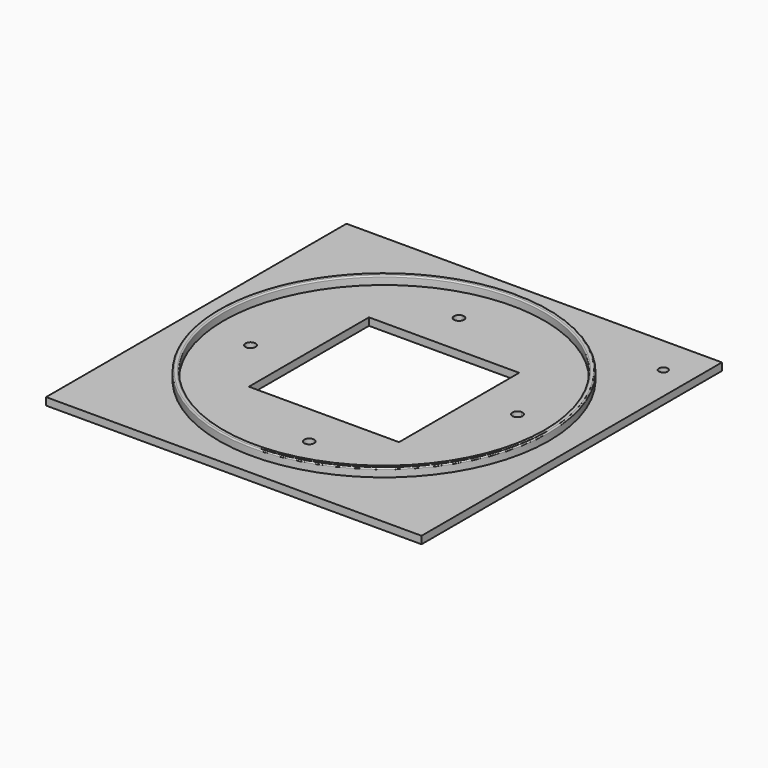
from build123d import *

# Parameters (mm, degrees)
F0_W     = 150
F0_H     = 150
F0_W_2   = 60
F0_H_2   = 60
F1_DEPTH = 3
F2_R     = 66
F2_R_2   = 64
F3_DEPTH = 3.3
F5_DEPTH = 2.3
F6_R     = 0.5
F7_R     = 0.5
F4_R     = 1.75
F8_DEPTH = 25


# Not quite as in the source:
# - a feature names something its author has since deleted; it is built from what else it names


with BuildPart() as f1:
    # F0 (on Top) → F1 (new body)
    with BuildSketch(Plane.XY):
        Rectangle(F0_W, F0_H)
        Rectangle(F0_W_2, F0_H_2, mode=Mode.SUBTRACT)
    extrude(amount=F1_DEPTH)

    # F2 (on face) → F3 (join)
    with BuildSketch(Plane.XY.offset(3)):
        Circle(F2_R)
        Circle(F2_R_2, mode=Mode.SUBTRACT)
    extrude(amount=F3_DEPTH)

    # F4 (on face) → F5 (cut)
    with BuildSketch(Plane.XY.offset(3)):
        with BuildLine():
            ThreePointArc((-49.1, -7.8), (-48.5142135624, -9.2142135624), (-47.1, -9.8))
            Line((-47.1, -9.8), (-47.1, -7.8))
            Line((-47.1, -7.8), (-49.1, -7.8))
        make_face()
        with BuildLine():
            Line((-47.1, -7.8), (-47.1, -9.8))
            ThreePointArc((-47.1, -9.8), (-45.6857864376, -9.2142135624), (-45.1, -7.8))
            ThreePointArc((-45.1, -7.8), (-47.1, -5.8), (-49.1, -7.8))
            Line((-49.1, -7.8), (-47.1, -7.8))
        make_face()
        with BuildLine():
            Line((-7.8, 47.2), (-9.8, 47.2))
            ThreePointArc((-9.8, 47.2), (-7.8, 45.2), (-5.8, 47.2))
            ThreePointArc((-5.8, 47.2), (-6.3857864376, 48.6142135624), (-7.8, 49.2))
            Line((-7.8, 49.2), (-7.8, 47.2))
        make_face()
        with BuildLine():
            ThreePointArc((-7.8, 49.2), (-9.2142135624, 48.6142135624), (-9.8, 47.2))
            Line((-9.8, 47.2), (-7.8, 47.2))
            Line((-7.8, 47.2), (-7.8, 49.2))
        make_face()
        with BuildLine():
            Line((47.1, 7.8), (47.1, 9.8))
            ThreePointArc((47.1, 9.8), (45.6857864376, 6.3857864376), (49.1, 7.8))
            Line((49.1, 7.8), (47.1, 7.8))
        make_face()
        with BuildLine():
            ThreePointArc((49.1, 7.8), (48.5142135624, 9.2142135624), (47.1, 9.8))
            Line((47.1, 9.8), (47.1, 7.8))
            Line((47.1, 7.8), (49.1, 7.8))
        make_face()
        with BuildLine():
            ThreePointArc((9.8, -47.1), (6.3857864376, -45.6857864376), (7.8, -49.1))
            Line((7.8, -49.1), (7.8, -47.1))
            Line((7.8, -47.1), (9.8, -47.1))
        make_face()
        with BuildLine():
            Line((7.8, -47.1), (7.8, -49.1))
            ThreePointArc((7.8, -49.1), (9.2142135624, -48.5142135624), (9.8, -47.1))
            Line((9.8, -47.1), (7.8, -47.1))
        make_face()
    extrude(amount=-F5_DEPTH, mode=Mode.SUBTRACT)

    # F6
    f6_edges = [f1.edges().sort_by_distance(p)[0] for p in [
        (-66, 0, 6.3),
    ]]
    fillet(f6_edges, radius=F6_R)

    # F7
    f7_edges = [f1.edges().sort_by_distance(p)[0] for p in [
        (-64, 0, 6.3),
    ]]
    fillet(f7_edges, radius=F7_R)

    # F4 (on face) → F8 (cut)
    with BuildSketch(Plane.XY.offset(3)):
        with Locations((63.9, 59.6)):
            Circle(F4_R)
    extrude(amount=-F8_DEPTH, mode=Mode.SUBTRACT)


solid = f1.part
